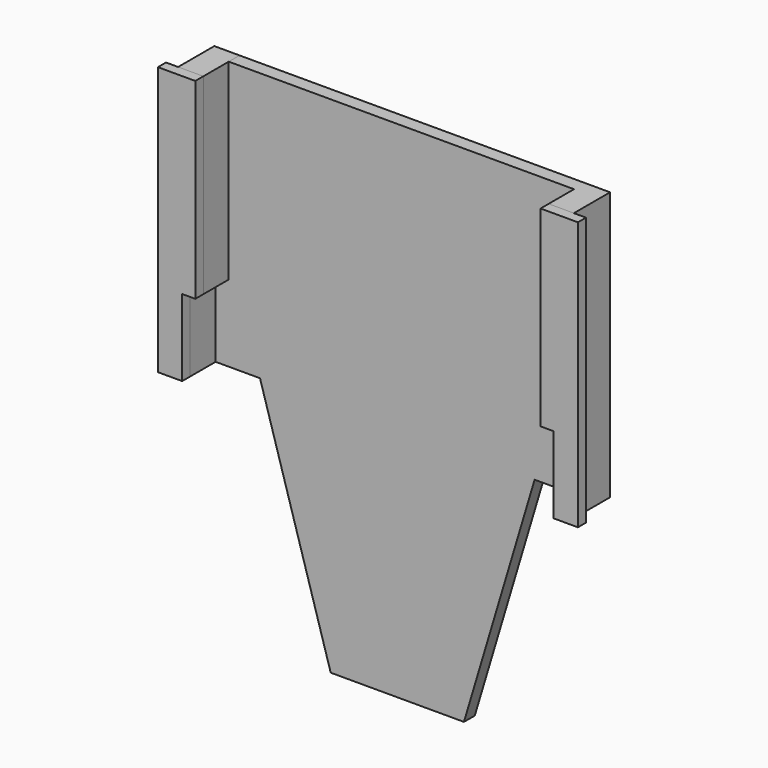
from build123d import *

# Parameters (mm, degrees)
F0_W     = 3
F0_H     = 66.5
F1_DEPTH = 2.5
F2_DEPTH = 11.2
F4_DEPTH = 3.35


with BuildPart() as f1:
    # F0 (on Front) → F1 (new body)
    with BuildSketch(Plane.XZ):
        with Locations((-107.2585358843, -14.25)):
            Rectangle(F0_W, F0_H)
        Polygon((-99.5085358843, 19), (-105.7585358843, 19), (-105.7585358843, -47.5), (-102.7585358843, -47.5), (-102.7585358843, -28.5), (-99.5085358843, -28.5), align=None)
    extrude(amount=F1_DEPTH)


with BuildPart() as f1b:
    # F0 (on Front) → F1, piece 2 (new body)
    with BuildSketch(Plane.XZ):
        with Locations((-6.2585358843, -14.25)):
            Rectangle(F0_W, F0_H)
        Polygon((-13.5085358843, 19), (-14.0085358843, 19), (-14.0085358843, -28.5), (-10.7585358843, -28.5), (-10.7585358843, -47.5), (-7.7585358843, -47.5), (-7.7585358843, 19), align=None)
    extrude(amount=F1_DEPTH)


with BuildPart() as f2:
    # F0 (on Front) → F2 (new body)
    with BuildSketch(Plane.XZ):
        Polygon((-99.5085358843, 19), (-105.7585358843, 19), (-105.7585358843, -47.5), (-102.7585358843, -47.5), (-102.7585358843, -28.5), (-99.5085358843, -28.5), align=None)
    extrude(amount=-F2_DEPTH)


with BuildPart() as f2b:
    # F0 (on Front) → F2, piece 2 (new body)
    with BuildSketch(Plane.XZ):
        Polygon((-13.5085358843, 19), (-14.0085358843, 19), (-14.0085358843, -28.5), (-10.7585358843, -28.5), (-10.7585358843, -47.5), (-7.7585358843, -47.5), (-7.7585358843, 19), align=None)
    extrude(amount=-F2_DEPTH)

    # F3 (on face) → F4 (join)
    with BuildSketch(Plane(origin=(0, 11.2, 0), x_dir=(-1, 0, 0), z_dir=(0, 1, 0))):
        Polygon((91.7585358843, -47.5), (102.7585358843, -47.5), (102.7585358843, -28.5), (99.5085358843, -28.5), (99.5085358843, 19), (57.7585358843, 19), (57.7585358843, -47.5), align=None)
        Polygon((74.2585358843, -106), (91.7585358843, -47.5), (57.7585358843, -47.5), (57.7585358843, -106), align=None)
        Polygon((57.7585358843, -106), (57.7585358843, -47.5), (23.7585358843, -47.5), (41.2585358843, -106), align=None)
        Polygon((23.7585358843, -47.5), (57.7585358843, -47.5), (57.7585358843, 19), (9.7585358843, 19), (9.7585358843, -47.5), align=None)
    extrude(amount=-F4_DEPTH)


solid = Compound([f1.part, f1b.part, f2.part, f2b.part])
